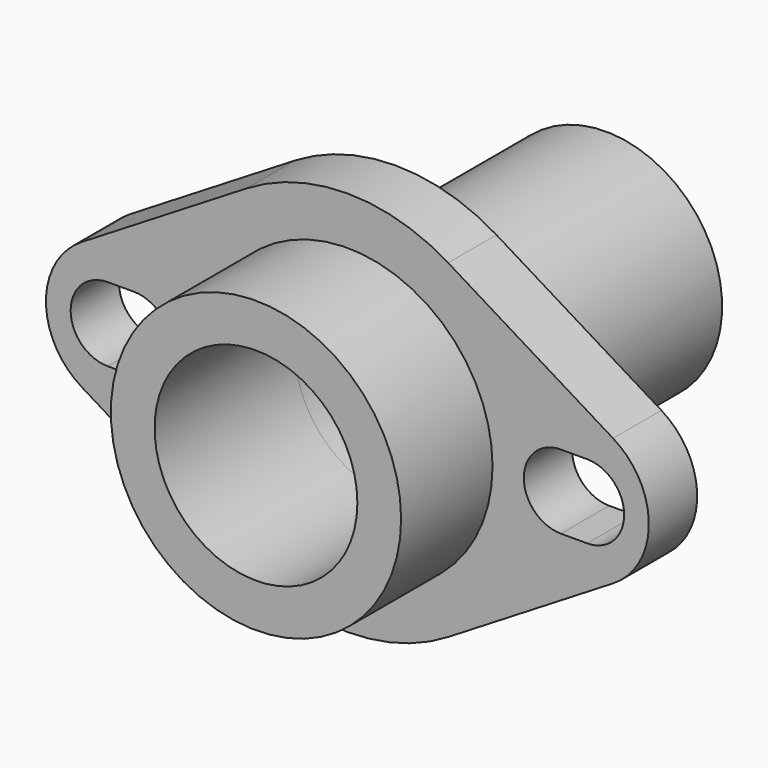
from build123d import *

# Parameters (mm, degrees)
F0_R     = 9.8044
F1_DEPTH = 5.842
F3_DEPTH = 5.843
F4_R     = 14.0335
F4_R_2   = 9.8044
F5_DEPTH = 11.049
F6_R     = 11.2395
F6_R_2   = 9.8044
F7_DEPTH = 25.4


# Not quite as in the source:
# - a pattern or mirror of a feature is missing from the dataset's text; its kind, count and spacing are read off the source's solid


with BuildPart() as f1:
    # F0 (on Front) → F1 (new body)
    with BuildSketch(Plane.XZ):
        with BuildLine():
            Line((25.6843695652, 6.1756276837), (9.7403478261, 15.9266187632))
            ThreePointArc((9.7403478261, 15.9266187632), (0, 18.669), (-9.7403478261, 15.9266187632))
            Line((-9.7403478261, 15.9266187632), (-25.6843695652, 6.1756276837))
            ThreePointArc((-25.6843695652, 6.1756276837), (-29.1465, 0), (-25.6843695652, -6.1756276837))
            Line((-25.6843695652, -6.1756276837), (-9.7403478261, -15.9266187632))
            ThreePointArc((-9.7403478261, -15.9266187632), (0, -18.669), (9.7403478261, -15.9266187632))
            Line((9.7403478261, -15.9266187632), (25.6843695652, -6.1756276837))
            ThreePointArc((25.6843695652, -6.1756276837), (29.1465, 0), (25.6843695652, 6.1756276837))
        make_face()
        Circle(F0_R, mode=Mode.SUBTRACT)
    extrude(amount=F1_DEPTH)

    # F2 (on face) → F3 (cut, through all)
    with BuildSketch(Plane.XZ.offset(5.842)):
        with BuildLine():
            ThreePointArc((-23.1775, 3.5814), (-26.7589, 0), (-23.1775, -3.5814))
            Line((-23.1775, -3.5814), (-20.6375, -3.5814))
            ThreePointArc((-20.6375, -3.5814), (-17.0561, 0), (-20.6375, 3.5814))
            Line((-20.6375, 3.5814), (-23.1775, 3.5814))
        make_face()
    f3 = extrude(amount=-F3_DEPTH, mode=Mode.SUBTRACT)

    # F3_copies: F3 across plane
    add(f3.mirror(Plane(origin=(0, 0, 0), x_dir=(0, 0, 1), z_dir=(1, 0, 0))), mode=Mode.SUBTRACT)

    # F4 (on face) → F5 (join)
    with BuildSketch(Plane.XZ.offset(5.842)):
        Circle(F4_R)
        Circle(F4_R_2, mode=Mode.SUBTRACT)
    extrude(amount=F5_DEPTH)

    # F6 (on face) → F7 (join)
    with BuildSketch(Plane(origin=(0, 0, 0), x_dir=(-1, 0, 0), z_dir=(0, 1, 0))):
        Circle(F6_R)
        Circle(F6_R_2, mode=Mode.SUBTRACT)
    extrude(amount=F7_DEPTH)


solid = f1.part
